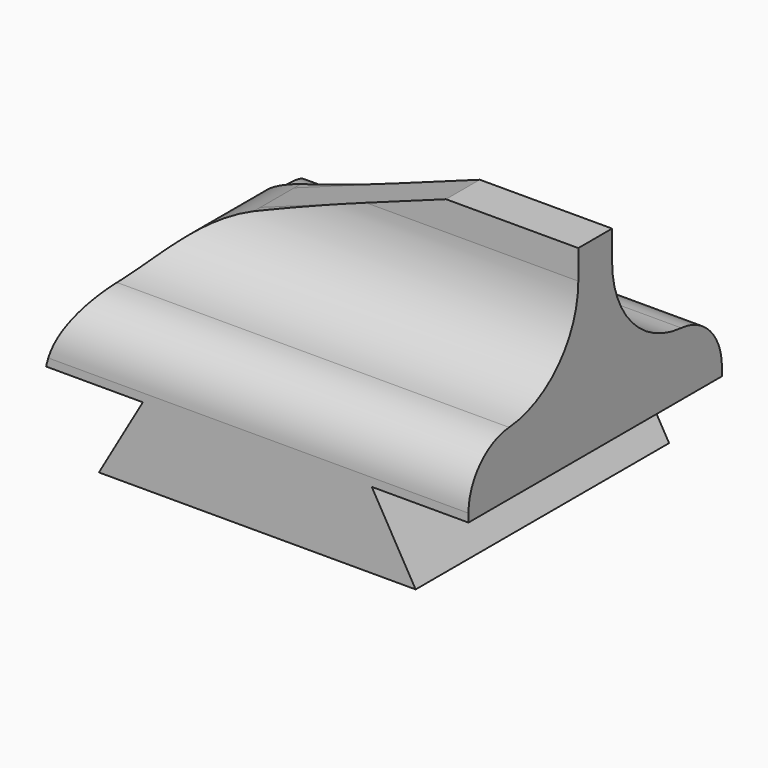
from build123d import *

# Parameters (mm, degrees)
F0_W         = 9.525
F0_H         = 9.525
F1_DEPTH     = 2.286
F2_T1_DEPTH  = 21.3619144247
F3_W         = 2.9083
F3_H         = 9.525
F3_W_2       = 6.8834
F4_DEPTH     = 1.905
F5_R         = 1.6556676611
F6_W         = 12.7
F6_H         = 1.27
F7_DEPTH     = 3.683
F8_SIZE2     = 8.7232408068
F8_SIZE      = 3.175
F9_T4_DEPTH  = 12.7
F9_T9_DEPTH  = 12.7
F10_T1_DEPTH = 20.6733949541


# Not quite as in the source:
# - a fillet or chamfer that OpenCascade refuses, or shapes differently, is made with other operations: its cross-section is extruded or revolved along the edge and cut away or added


with BuildPart() as f1:
    # F0 (on Top) → F1 (new body)
    with BuildSketch(Plane.XY):
        Rectangle(F0_W, F0_H)
    extrude(amount=F1_DEPTH)

    # F2: chamfer of 1.3208 x 2.2876927066 on 2 edges, made by hand

    # F2_s2 → F2_t1 (cut)
    with BuildSketch(Plane.XZ.offset(-10.6809572123)):
        Polygon((-4.7625, -0.0016927066), (-3.4417, 2.286), (-4.7625, 2.286), align=None)
        Polygon((4.7625, -0.0016927066), (3.4417, 2.286), (4.7625, 2.286), align=None)
    extrude(amount=F2_T1_DEPTH, mode=Mode.SUBTRACT)

    # F3 (on face) → F4 (join)
    with BuildSketch(Plane.XY.offset(2.286)):
        with Locations((4.89585, 0)):
            Rectangle(F3_W, F3_H)
        Rectangle(F3_W_2, F3_H)
        with Locations((-4.89585, 0)):
            Rectangle(F3_W, F3_H)
    extrude(amount=F4_DEPTH)

    # F5
    f5_edges = [f1.edges().sort_by_distance(p)[0] for p in [
        (0, 4.7625, 4.191),
        (0, -4.7625, 4.191),
    ]]
    fillet(f5_edges, radius=F5_R)

    # F6 (on face) → F7 (join)
    with BuildSketch(Plane.XY.offset(4.191)):
        Rectangle(F6_W, F6_H)
    extrude(amount=F7_DEPTH)

    # F8
    f8_edges = [f1.edges().sort_by_distance(p)[0] for p in [
        (-6.35, 0, 7.874),
    ]]
    f8_side = f1.faces().sort_by_distance((-6.35, 0, 3.810575))[0]
    chamfer(f8_edges, length=F8_SIZE, length2=F8_SIZE2, reference=f8_side)

    # F9: fillet of radius 2.8207671263 on 2 edges, made by hand


with BuildPart() as f9_tool2:
    # F9_s3 → F9_t4 (new body)
    with BuildSketch(Plane.YZ.offset(-6.35)):
        with BuildLine():
            ThreePointArc((-0.635, 6.9981468006), (-1.3849039981, 5.0828783899), (-3.235890411, 4.1859623453))
            Line((-3.235890411, 4.1859623453), (-3.2139027394, 3.9047438998))
            ThreePointArc((-3.2139027394, 3.9047438998), (-3.1068323389, 3.9089232874), (-0.635, 3.9089232874))
            Line((-0.635, 3.9089232874), (-0.3529232874, 4.191))
            Line((-0.3529232874, 4.191), (-0.3529232874, 6.9981468006))
            Line((-0.3529232874, 6.9981468006), (-0.635, 6.9981468006))
        make_face()
    extrude(amount=F9_T4_DEPTH)

    split(bisect_by=Plane(origin=(-2.2530383821, 0, 6.1901720799), x_dir=(0, 1, 0), z_dir=(0.3420201433, 0, -0.9396926208)), keep=Keep.TOP)


with BuildPart() as f1_1:
    add(f1.part)

    # F9_t1: union F9_tool2
    add(f9_tool2.part)


with BuildPart() as f9_tool7:
    # F9_s8 → F9_t9 (new body)
    with BuildSketch(Plane.YZ.offset(6.35)):
        with BuildLine():
            ThreePointArc((0.635, 6.9981468006), (1.3849039981, 5.0828783899), (3.235890411, 4.1859623453))
            Line((3.235890411, 4.1859623453), (3.2139027394, 3.9047438998))
            ThreePointArc((3.2139027394, 3.9047438998), (3.1068323389, 3.9089232874), (0.635, 3.9089232874))
            Line((0.635, 3.9089232874), (0.3529232874, 4.191))
            Line((0.3529232874, 4.191), (0.3529232874, 6.9981468006))
            Line((0.3529232874, 6.9981468006), (0.635, 6.9981468006))
        make_face()
    extrude(amount=-F9_T9_DEPTH)

    split(bisect_by=Plane(origin=(-2.2530383821, 0, 6.1901720799), x_dir=(0, 1, 0), z_dir=(0.3420201433, 0, -0.9396926208)), keep=Keep.TOP)


with BuildPart() as f1_2:
    add(f1_1.part)

    # F9_t6: union F9_tool7
    add(f9_tool7.part)

    # F10: fillet of radius 5.08 on 1 edges, made by hand

    # F10_s2 → F10_t1 (cut)
    with BuildSketch(Plane.XZ.offset(-10.336697477)):
        with BuildLine():
            ThreePointArc((-6.3503887376, 2.2860942499), (-5.1990968175, 4.4769990033), (-3.1494899918, 5.8643160486))
            Line((-3.1494899918, 5.8643160486), (-3.3233118727, 6.3418877414))
            ThreePointArc((-3.3233118727, 6.3418877414), (-4.9234984728, 5.7590417786), (-6.5238218809, 5.1765716928))
            Line((-6.5238218809, 5.1765716928), (-6.8582211803, 4.699))
            ThreePointArc((-6.8582211803, 4.699), (-6.8582211803, 3.492547125), (-6.8443004931, 2.4058437629))
            Line((-6.8443004931, 2.4058437629), (-6.3503887376, 2.2860942499))
        make_face()
    extrude(amount=F10_T1_DEPTH, mode=Mode.SUBTRACT)


solid = f1_2.part
